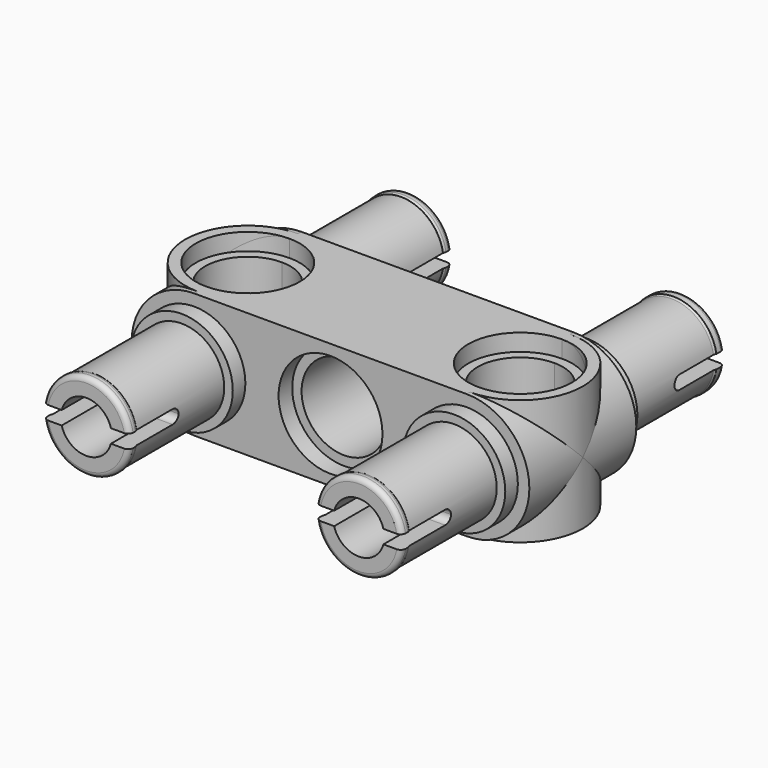
from build123d import *

# Parameters (mm, degrees)
F0_R      = 3.05
F0_R_2    = 3
F0_R_3    = 2.499
F1_DEPTH  = 3.925
F2_DEPTH  = 4.85
F3_DEPTH  = 11.25
F4_R      = 2.55
F5_DEPTH  = 0.6
F6_R      = 2.55
F7_DEPTH  = 0.6
F8_R      = 2.55
F9_DEPTH  = 0.6
F10_R     = 2.55
F11_DEPTH = 0.6
F12_R     = 1.5
F13_DEPTH = 7.925
F14_R     = 1.5
F15_DEPTH = 7.925
F16_R     = 1.5
F17_DEPTH = 7.925
F18_R     = 1.5
F19_DEPTH = 7.925
F21_R     = 3.675
F21_R_2   = 3.05
F22_DEPTH = 7.35
F23_DEPTH = 7.3510001
F24_DEPTH = 1
F26_DEPTH = 1
F27_R     = 3.05
F27_R_2   = 2.499
F28_DEPTH = 1
F29_R     = 3.05
F29_R_2   = 2.499
F30_DEPTH = 1
F31_R     = 2.499
F32_DEPTH = 5.35
F33_R     = 2.499
F34_DEPTH = 5.35
F35_W     = 3.65
F35_H     = 0.8
F36_DEPTH = 12.5
F37_R     = 0.3999


# Not quite as in the source:
# - a fillet or chamfer that OpenCascade refuses, or shapes differently, is made with other operations: its cross-section is extruded or revolved along the edge and cut away or added
# - a fillet or chamfer is up to 0.001 mm smaller than in the source, because OpenCascade refuses the exact size


with BuildPart() as f1:
    # F0 (on Front) → F1 (new body, symmetric)
    with BuildSketch(Plane.XZ):
        with BuildLine():
            ThreePointArc((8, -3.675), (4.325, 0), (8, 3.675))
            Line((8, 3.675), (-8.0000000262, 3.675))
            ThreePointArc((-8.0000000262, 3.675), (-5.4013825884, 2.5986174301), (-4.325, 0))
            ThreePointArc((-4.325, 0), (-5.4013825791, -2.5986174209), (-8, -3.675))
            Line((-8, -3.675), (8, -3.675))
        make_face()
        Circle(F0_R, mode=Mode.SUBTRACT)
        with BuildLine():
            ThreePointArc((-4.325, 0), (-5.4013825884, 2.5986174301), (-8.0000000262, 3.675))
            ThreePointArc((-8.0000000262, 3.675), (-10.5986174301, 2.5986174116), (-11.675, 0))
            ThreePointArc((-11.675, 0), (-10.5986174209, -2.5986174209), (-8, -3.675))
            ThreePointArc((-8, -3.675), (-5.4013825791, -2.5986174209), (-4.325, 0))
        make_face()
        with Locations((-8, 0)):
            Circle(F0_R_2, mode=Mode.SUBTRACT)
        with BuildLine():
            ThreePointArc((11.675, 0), (10.5986174209, 2.5986174209), (8, 3.675))
            ThreePointArc((8, 3.675), (4.325, 0), (8, -3.675))
            ThreePointArc((8, -3.675), (10.5986174209, -2.5986174209), (11.675, 0))
        make_face()
        with Locations((8, 0)):
            Circle(F0_R_2, mode=Mode.SUBTRACT)
        Circle(F0_R)
        Circle(F0_R_3, mode=Mode.SUBTRACT)
    extrude(amount=F1_DEPTH, both=True)

    # F0 (on Front) → F2 (join, symmetric)
    with BuildSketch(Plane.XZ):
        with Locations((-8, 0)):
            Circle(F0_R_2)
        with Locations((-8, 0)):
            Circle(F0_R_3, mode=Mode.SUBTRACT)
        with Locations((8, 0)):
            Circle(F0_R_2)
        with Locations((8, 0)):
            Circle(F0_R_3, mode=Mode.SUBTRACT)
    extrude(amount=F2_DEPTH, both=True)

    # F0 (on Front) → F3 (join, symmetric)
    with BuildSketch(Plane.XZ):
        with Locations((-8, 0)):
            Circle(F0_R_3)
        with Locations((8, 0)):
            Circle(F0_R_3)
    extrude(amount=F3_DEPTH, both=True)

    # F4 (on face) → F5 (join)
    with BuildSketch(Plane.XZ.offset(11.25)):
        with Locations((-8, 0)):
            Circle(F4_R)
    extrude(amount=F5_DEPTH)

    # F6 (on face) → F7 (join)
    with BuildSketch(Plane.XZ.offset(11.25)):
        with Locations((8, 0)):
            Circle(F6_R)
    extrude(amount=F7_DEPTH)

    # F8 (on face) → F9 (join)
    with BuildSketch(Plane(origin=(0, 11.25, 0), x_dir=(-1, 0, 0), z_dir=(0, 1, 0))):
        with Locations((8, 0)):
            Circle(F8_R)
    extrude(amount=F9_DEPTH)

    # F10 (on face) → F11 (join)
    with BuildSketch(Plane(origin=(0, 11.25, 0), x_dir=(-1, 0, 0), z_dir=(0, 1, 0))):
        with Locations((-8, 0)):
            Circle(F10_R)
    extrude(amount=F11_DEPTH)

    # F12 (on face) → F13 (cut, through all)
    with BuildSketch(Plane(origin=(0, 11.85, 0), x_dir=(-1, 0, 0), z_dir=(0, 1, 0))):
        with Locations((8, 0)):
            Circle(F12_R)
    extrude(amount=-F13_DEPTH, mode=Mode.SUBTRACT)

    # F14 (on face) → F15 (cut, through all)
    with BuildSketch(Plane(origin=(0, 11.85, 0), x_dir=(-1, 0, 0), z_dir=(0, 1, 0))):
        with Locations((-8, 0)):
            Circle(F14_R)
    extrude(amount=-F15_DEPTH, mode=Mode.SUBTRACT)

    # F16 (on face) → F17 (cut, through all)
    with BuildSketch(Plane.XZ.offset(11.85)):
        with Locations((8, 0)):
            Circle(F16_R)
    extrude(amount=-F17_DEPTH, mode=Mode.SUBTRACT)

    # F18 (on face) → F19 (cut, through all)
    with BuildSketch(Plane.XZ.offset(11.85)):
        with Locations((-8, 0)):
            Circle(F18_R)
    extrude(amount=-F19_DEPTH, mode=Mode.SUBTRACT)

    # F20: fillet of radius 0.3 on 8 edges, made by hand

    # F20_s1 → F20_t2 (revolve)
    with BuildSketch(Plane.XY):
        with BuildLine():
            ThreePointArc((10.5496677818, 11.2502227803), (10.5116494739, 11.1700982799), (10.4986, 11.0823769112))
            Line((10.4986, 11.0823769112), (10.4684634315, 11.0823769112))
            ThreePointArc((10.4684634315, 11.0823769112), (10.4688634315, 11.1661884556), (10.4688634315, 11.25))
            Line((10.4688634315, 11.25), (10.499, 11.2801365685))
            ThreePointArc((10.499, 11.2801365685), (10.5243338909, 11.2801365685), (10.5246379915, 11.2670073673))
            Line((10.5246379915, 11.2670073673), (10.5496677818, 11.2502227803))
        make_face()
    revolve(axis=Axis((8, 11.25, 0), (0, -1, 0)))

    # F20_s3 → F20_t4 (revolve, cut)
    with BuildSketch(Plane.XY):
        with BuildLine():
            ThreePointArc((-5.4496, -11.5490343146), (-5.5378679656, -11.7621320344), (-5.7509656854, -11.8504))
            Line((-5.7509656854, -11.8504), (-5.7509656854, -11.8805365685))
            ThreePointArc((-5.7509656854, -11.8805365685), (-5.6004828427, -11.8801365685), (-5.45, -11.8801365685))
            Line((-5.45, -11.8801365685), (-5.4198634315, -11.85))
            ThreePointArc((-5.4198634315, -11.85), (-5.4198634315, -11.6995171573), (-5.4194634315, -11.5490343146))
            Line((-5.4194634315, -11.5490343146), (-5.4496, -11.5490343146))
        make_face()
    revolve(axis=Axis((-8, -11.85, 0), (0, -1, 0)), mode=Mode.SUBTRACT)

    # F20_s5 → F20_t6 (revolve, cut)
    with BuildSketch(Plane.XY):
        with BuildLine():
            ThreePointArc((-5.5006677818, -11.2497772197), (-5.4626494739, -11.3299017201), (-5.4496, -11.4176230888))
            Line((-5.4496, -11.4176230888), (-5.4194634315, -11.4176230888))
            ThreePointArc((-5.4194634315, -11.4176230888), (-5.4198634315, -11.3338115444), (-5.4198634315, -11.25))
            Line((-5.4198634315, -11.25), (-5.45, -11.2198634315))
            ThreePointArc((-5.45, -11.2198634315), (-5.4753338909, -11.2198634315), (-5.4756379915, -11.2329926327))
            Line((-5.4756379915, -11.2329926327), (-5.5006677818, -11.2497772197))
        make_face()
    revolve(axis=Axis((-8, -11.25, 0), (0, -1, 0)), mode=Mode.SUBTRACT)

    # F20_s7 → F20_t8 (revolve, cut)
    with BuildSketch(Plane.XY):
        with BuildLine():
            ThreePointArc((10.5504, -11.5490343146), (10.4621320344, -11.7621320344), (10.2490343146, -11.8504))
            Line((10.2490343146, -11.8504), (10.2490343146, -11.8805365685))
            ThreePointArc((10.2490343146, -11.8805365685), (10.3995171573, -11.8801365685), (10.55, -11.8801365685))
            Line((10.55, -11.8801365685), (10.5801365685, -11.85))
            ThreePointArc((10.5801365685, -11.85), (10.5801365685, -11.6995171573), (10.5805365685, -11.5490343146))
            Line((10.5805365685, -11.5490343146), (10.5504, -11.5490343146))
        make_face()
    revolve(axis=Axis((8, -11.85, 0), (0, -1, 0)), mode=Mode.SUBTRACT)

    # F20_s9 → F20_t10 (revolve, cut)
    with BuildSketch(Plane.XY):
        with BuildLine():
            ThreePointArc((10.4993322182, -11.2497772197), (10.5373505261, -11.3299017201), (10.5504, -11.4176230888))
            Line((10.5504, -11.4176230888), (10.5805365685, -11.4176230888))
            ThreePointArc((10.5805365685, -11.4176230888), (10.5801365685, -11.3338115444), (10.5801365685, -11.25))
            Line((10.5801365685, -11.25), (10.55, -11.2198634315))
            ThreePointArc((10.55, -11.2198634315), (10.5246661091, -11.2198634315), (10.5243620085, -11.2329926327))
            Line((10.5243620085, -11.2329926327), (10.4993322182, -11.2497772197))
        make_face()
    revolve(axis=Axis((8, -11.25, 0), (0, -1, 0)), mode=Mode.SUBTRACT)

    # F20_s11 → F20_t12 (revolve, cut)
    with BuildSketch(Plane.XY):
        with BuildLine():
            ThreePointArc((-10.5504, 11.5490343146), (-10.4621320344, 11.7621320344), (-10.2490343146, 11.8504))
            Line((-10.2490343146, 11.8504), (-10.2490343146, 11.8805365685))
            ThreePointArc((-10.2490343146, 11.8805365685), (-10.3995171573, 11.8801365685), (-10.55, 11.8801365685))
            Line((-10.55, 11.8801365685), (-10.5801365685, 11.85))
            ThreePointArc((-10.5801365685, 11.85), (-10.5801365685, 11.6995171573), (-10.5805365685, 11.5490343146))
            Line((-10.5805365685, 11.5490343146), (-10.5504, 11.5490343146))
        make_face()
    revolve(axis=Axis((-8, 11.85, 0), (0, 1, 0)), mode=Mode.SUBTRACT)

    # F20_s13 → F20_t14 (revolve, cut)
    with BuildSketch(Plane.XY):
        with BuildLine():
            ThreePointArc((-10.4993322182, 11.2497772197), (-10.5373505261, 11.3299017201), (-10.5504, 11.4176230888))
            Line((-10.5504, 11.4176230888), (-10.5805365685, 11.4176230888))
            ThreePointArc((-10.5805365685, 11.4176230888), (-10.5801365685, 11.3338115444), (-10.5801365685, 11.25))
            Line((-10.5801365685, 11.25), (-10.55, 11.2198634315))
            ThreePointArc((-10.55, 11.2198634315), (-10.5246661091, 11.2198634315), (-10.5243620085, 11.2329926327))
            Line((-10.5243620085, 11.2329926327), (-10.4993322182, 11.2497772197))
        make_face()
    revolve(axis=Axis((-8, 11.25, 0), (0, 1, 0)), mode=Mode.SUBTRACT)

    # F20_s15 → F20_t16 (revolve, cut)
    with BuildSketch(Plane.XY):
        with BuildLine():
            ThreePointArc((5.4496, 11.5490343146), (5.5378679656, 11.7621320344), (5.7509656854, 11.8504))
            Line((5.7509656854, 11.8504), (5.7509656854, 11.8805365685))
            ThreePointArc((5.7509656854, 11.8805365685), (5.6004828427, 11.8801365685), (5.45, 11.8801365685))
            Line((5.45, 11.8801365685), (5.4198634315, 11.85))
            ThreePointArc((5.4198634315, 11.85), (5.4198634315, 11.6995171573), (5.4194634315, 11.5490343146))
            Line((5.4194634315, 11.5490343146), (5.4496, 11.5490343146))
        make_face()
    revolve(axis=Axis((8, 11.85, 0), (0, 1, 0)), mode=Mode.SUBTRACT)

    # F21 (on face) → F22 (join, through all)
    with BuildSketch(Plane.XY.offset(3.675)):
        with Locations((-8, 0)):
            Circle(F21_R)
        with Locations((-8, 0)):
            Circle(F21_R_2, mode=Mode.SUBTRACT)
        with Locations((8, 0)):
            Circle(F21_R)
        with Locations((8, 0)):
            Circle(F21_R_2, mode=Mode.SUBTRACT)
    extrude(amount=-F22_DEPTH)

    # F21 (on face) → F23 (cut, through all)
    with BuildSketch(Plane.XY.offset(3.675)):
        with BuildLine():
            Line((-8.0000000262, -2.499), (-8.0000000262, 2.499))
            ThreePointArc((-8.0000000262, 2.499), (-10.499, 0), (-8.0000000262, -2.499))
        make_face()
        with BuildLine():
            ThreePointArc((-5.501, 0), (-6.2329401631, 1.7670598554), (-8.0000000262, 2.499))
            Line((-8.0000000262, 2.499), (-8.0000000262, -2.499))
            ThreePointArc((-8.0000000262, -2.499), (-6.2329401631, -1.7670598554), (-5.501, 0))
        make_face()
        with BuildLine():
            ThreePointArc((10.499, 0), (9.7670598462, 1.7670598462), (8, 2.499))
            Line((8, 2.499), (8, -2.499))
            ThreePointArc((8, -2.499), (9.7670598462, -1.7670598462), (10.499, 0))
        make_face()
        with BuildLine():
            Line((8, -2.499), (8, 2.499))
            ThreePointArc((8, 2.499), (5.501, 0), (8, -2.499))
        make_face()
    extrude(amount=-F23_DEPTH, mode=Mode.SUBTRACT)

    # F21 (on face) → F24 (cut)
    with BuildSketch(Plane.XY.offset(3.675)):
        with BuildLine():
            ThreePointArc((-4.95, 0), (-5.8433243266, 2.1566756919), (-8.0000000262, 3.05))
            Line((-8.0000000262, 3.05), (-8.0000000262, 2.499))
            ThreePointArc((-8.0000000262, 2.499), (-6.2329401631, 1.7670598554), (-5.501, 0))
            ThreePointArc((-5.501, 0), (-6.2329401631, -1.7670598554), (-8.0000000262, -2.499))
            Line((-8.0000000262, -2.499), (-8.0000000262, -3.05))
            ThreePointArc((-8.0000000262, -3.05), (-5.8433243266, -2.1566756919), (-4.95, 0))
        make_face()
        with BuildLine():
            ThreePointArc((11.05, 0), (10.1566756826, 2.1566756826), (8, 3.05))
            Line((8, 3.05), (8, 2.499))
            ThreePointArc((8, 2.499), (9.7670598462, 1.7670598462), (10.499, 0))
            ThreePointArc((10.499, 0), (9.7670598462, -1.7670598462), (8, -2.499))
            Line((8, -2.499), (8, -3.05))
            ThreePointArc((8, -3.05), (10.1566756826, -2.1566756826), (11.05, 0))
        make_face()
        with BuildLine():
            Line((8, 2.499), (8, 3.05))
            ThreePointArc((8, 3.05), (4.95, 0), (8, -3.05))
            Line((8, -3.05), (8, -2.499))
            ThreePointArc((8, -2.499), (5.501, 0), (8, 2.499))
        make_face()
        with BuildLine():
            Line((-8.0000000262, 2.499), (-8.0000000262, 3.05))
            ThreePointArc((-8.0000000262, 3.05), (-11.05, 0), (-8.0000000262, -3.05))
            Line((-8.0000000262, -3.05), (-8.0000000262, -2.499))
            ThreePointArc((-8.0000000262, -2.499), (-10.499, 0), (-8.0000000262, 2.499))
        make_face()
    extrude(amount=-F24_DEPTH, mode=Mode.SUBTRACT)

    # F25 (on face) → F26 (cut)
    with BuildSketch(Plane(origin=(0, 0, -3.675), x_dir=(1, 0, 0), z_dir=(0, 0, -1))):
        with BuildLine():
            ThreePointArc((-8, -3.05), (-5.8433243174, -2.1566756826), (-4.95, 0))
            ThreePointArc((-4.95, 0), (-5.8433243174, 2.1566756826), (-8, 3.05))
            Line((-8, 3.05), (-8, 2.499))
            ThreePointArc((-8.0000000131, 2.499), (-6.2329401584, 1.7670598508), (-5.501, 0))
            ThreePointArc((-5.501, 0), (-6.2329401538, -1.7670598462), (-8, -2.499))
            Line((-8, -2.499), (-8, -3.05))
        make_face()
        with BuildLine():
            Line((-8, 2.499), (-8, 3.05))
            ThreePointArc((-8, 3.05), (-11.05, 0), (-8, -3.05))
            Line((-8, -3.05), (-8, -2.499))
            ThreePointArc((-8, -2.499), (-10.499, -6.5e-09), (-8.0000000131, 2.499))
        make_face()
        with BuildLine():
            ThreePointArc((8, 2.499), (9.7670598462, 1.7670598462), (10.499, 0))
            ThreePointArc((10.499, 0), (9.7670598462, -1.7670598462), (8, -2.499))
            Line((8, -2.499), (8, -3.05))
            ThreePointArc((8, -3.05), (10.1566756826, -2.1566756826), (11.05, 0))
            ThreePointArc((11.05, 0), (10.1566756826, 2.1566756826), (8, 3.05))
            Line((8, 3.05), (8, 2.499))
        make_face()
        with BuildLine():
            ThreePointArc((8, -2.499), (5.501, 0), (8, 2.499))
            Line((8, 2.499), (8, 3.05))
            ThreePointArc((8, 3.05), (4.95, 0), (8, -3.05))
            Line((8, -3.05), (8, -2.499))
        make_face()
    extrude(amount=-F26_DEPTH, mode=Mode.SUBTRACT)

    # F27 (on face) → F28 (cut)
    with BuildSketch(Plane(origin=(0, 3.925, 0), x_dir=(-1, 0, 0), z_dir=(0, 1, 0))):
        Circle(F27_R)
        Circle(F27_R_2, mode=Mode.SUBTRACT)
    extrude(amount=-F28_DEPTH, mode=Mode.SUBTRACT)

    # F29 (on face) → F30 (cut)
    with BuildSketch(Plane.XZ.offset(3.925)):
        Circle(F29_R)
        Circle(F29_R_2, mode=Mode.SUBTRACT)
    extrude(amount=-F30_DEPTH, mode=Mode.SUBTRACT)

    # F31 (on face) → F32 (join, through all)
    with BuildSketch(Plane.XY.offset(2.675)):
        with BuildLine():
            Line((10.5199206337, -1.7182840272), (10.5199206337, 1.7182840275))
            ThreePointArc((10.5199206338, 1.7182840275), (4.95, -1e-10), (10.519920634, -1.7182840272))
        make_face()
        with Locations((8, 0)):
            Circle(F31_R, mode=Mode.SUBTRACT)
        with BuildLine():
            ThreePointArc((10.519920634, -1.7182840272), (10.9144688996, -0.899094563), (11.05, 0))
            ThreePointArc((11.05, 0), (10.9144688996, 0.8990945631), (10.5199206338, 1.7182840275))
            Line((10.5199206337, 1.7182840275), (10.5199206337, -1.7182840272))
        make_face()
    extrude(amount=-F32_DEPTH)

    # F33 (on face) → F34 (join, through all)
    with BuildSketch(Plane.XY.offset(2.675)):
        with BuildLine():
            ThreePointArc((-10.5199206338, -1.7182840275), (-7.1009054369, -2.9144688996), (-4.95, 0))
            ThreePointArc((-4.95, 0), (-7.100905437, 2.9144688996), (-10.519920634, 1.7182840273))
            Line((-10.5199206337, 1.7182840272), (-10.5199206337, -1.7182840275))
        make_face()
        with Locations((-8, 0)):
            Circle(F33_R, mode=Mode.SUBTRACT)
        with BuildLine():
            Line((-10.5199206337, -1.7182840275), (-10.5199206337, 1.7182840272))
            ThreePointArc((-10.519920634, 1.7182840273), (-11.05, -1e-10), (-10.5199206338, -1.7182840275))
        make_face()
    extrude(amount=-F34_DEPTH)

    # F35 (on Right) → F36 (cut, symmetric)
    with BuildSketch(Plane.YZ):
        with Locations((10.025, 0)):
            Rectangle(F35_W, F35_H)
        with Locations((-10.025, 0)):
            Rectangle(F35_W, F35_H)
    extrude(amount=F36_DEPTH, both=True, mode=Mode.SUBTRACT)

    # F37 (radius 0.4 in the source; OpenCascade refuses exactly that, so slightly less here)
    f37_edges = [f1.edges().sort_by_distance(p)[0] for p in [
        (6.043769, 8.2, -0.4),
        (9.956231, 8.2, -0.4),
        (6.043769, 8.2, 0.4),
        (9.956231, 8.2, 0.4),
        (-6.043769, 8.2, 0.4),
        (-9.956231, 8.2, 0.4),
        (9.956231, -8.2, 0.4),
        (6.043769, -8.2, 0.4),
        (-6.043769, 8.2, -0.4),
        (-9.956231, 8.2, -0.4),
        (9.956231, -8.2, -0.4),
        (6.043769, -8.2, -0.4),
        (-6.043769, -8.2, -0.4),
        (-9.956231, -8.2, -0.4),
        (-6.043769, -8.2, 0.4),
        (-9.956231, -8.2, 0.4),
    ]]
    fillet(f37_edges, radius=F37_R)


solid = f1.part
